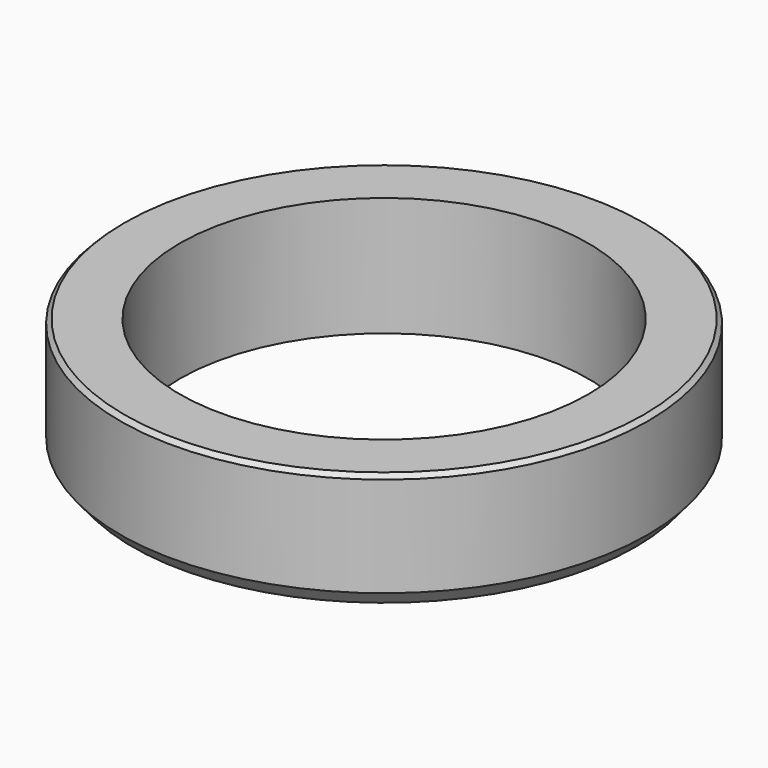
from build123d import *

# Parameters (mm, degrees)
F2_SIZE2 = 1.5748
F2_SIZE  = 1.5748
F4_DEPTH = 12.7
F5_R     = 76.2
F6_DEPTH = 44.451


with BuildPart() as f1:
    # F0 (on Front) → F1 (revolve)
    with BuildSketch(Plane.XZ):
        Polygon((98.425, 0), (0, 0), (0, -44.45), (93.726, -44.45), (98.425, -38.8499498684), align=None)
    revolve(axis=Axis((0, 0, -22.225), (0, 0, 1)))

    # F2
    f2_edges = [f1.edges().sort_by_distance(p)[0] for p in [
        (-98.425, 0, 0),
    ]]
    chamfer(f2_edges, length=F2_SIZE, length2=F2_SIZE2)

    # F3 (on face) → F4 (cut)
    with BuildSketch(Plane(origin=(0, 0, -44.45), x_dir=(1, 0, 0), z_dir=(0, 0, -1))):
        with BuildLine():
            ThreePointArc((59.6599475589, 65.9082745736), (59.7366637174, 59.7366637174), (65.9082745736, 59.6599475589))
            ThreePointArc((65.9082745736, 59.6599475589), (62.8617928475, 62.8617928475), (59.6599475589, 65.9082745736))
        make_face()
        with BuildLine():
            ThreePointArc((59.6599475589, 65.9082745736), (62.8617928475, 62.8617928475), (65.9082745736, 59.6599475589))
            ThreePointArc((65.9082745736, 59.6599475589), (66.923633243, 61.1198638129), (67.2813928475, 62.8617928475))
            ThreePointArc((67.2813928475, 62.8617928475), (64.5022179025, 66.9656775679), (59.6599475589, 65.9082745736))
        make_face()
        with BuildLine():
            ThreePointArc((90.2904059571, -23.0090131096), (89.343398088, -20.275157215), (86.9082138798, -18.7128928876))
            ThreePointArc((86.9082138798, -18.7128928876), (85.8708059571, -23.0090131096), (84.6211674612, -27.2482663209))
            ThreePointArc((84.6211674612, -27.2482663209), (88.5174984084, -26.5484881029), (90.2904059571, -23.0090131096))
        make_face()
        with BuildLine():
            ThreePointArc((84.6211674612, -27.2482663209), (85.8708059571, -23.0090131096), (86.9082138798, -18.7128928876))
            ThreePointArc((86.9082138798, -18.7128928876), (81.6018001752, -21.8651364579), (84.6211674612, -27.2482663209))
        make_face()
        with BuildLine():
            ThreePointArc((-18.5894131096, 85.8708059571), (-18.6203916237, 86.3931713593), (-18.7128928876, 86.9082138798))
            ThreePointArc((-18.7128928876, 86.9082138798), (-23.0090131096, 85.8708059571), (-27.2482663209, 84.6211674612))
            ThreePointArc((-27.2482663209, 84.6211674612), (-22.3777205201, 81.4965250075), (-18.5894131096, 85.8708059571))
        make_face()
        with BuildLine():
            ThreePointArc((-27.2482663209, 84.6211674612), (-23.0090131096, 85.8708059571), (-18.7128928876, 86.9082138798))
            ThreePointArc((-18.7128928876, 86.9082138798), (-24.1528897613, 90.139811739), (-27.2482663209, 84.6211674612))
        make_face()
        with BuildLine():
            ThreePointArc((27.4286131096, -85.8708059571), (27.3832940593, -85.2395133675), (27.2482663209, -84.6211674612))
            ThreePointArc((27.2482663209, -84.6211674612), (23.0090131096, -85.8708059571), (18.7128928876, -86.9082138798))
            ThreePointArc((18.7128928876, -86.9082138798), (23.5313785118, -90.259427443), (27.4286131096, -85.8708059571))
        make_face()
        with BuildLine():
            ThreePointArc((18.7128928876, -86.9082138798), (23.0090131096, -85.8708059571), (27.2482663209, -84.6211674612))
            ThreePointArc((27.2482663209, -84.6211674612), (21.8651364579, -81.6018001752), (18.7128928876, -86.9082138798))
        make_face()
        with BuildLine():
            ThreePointArc((-81.4512059571, 23.0090131096), (-82.3313309638, 25.6557055609), (-84.6211674612, 27.2482663209))
            ThreePointArc((-84.6211674612, 27.2482663209), (-85.8708059571, 23.0090131096), (-86.9082138798, 18.7128928876))
            ThreePointArc((-86.9082138798, 18.7128928876), (-83.1369500625, 19.5364209787), (-81.4512059571, 23.0090131096))
        make_face()
        with BuildLine():
            ThreePointArc((-86.9082138798, 18.7128928876), (-85.8708059571, 23.0090131096), (-84.6211674612, 27.2482663209))
            ThreePointArc((-84.6211674612, 27.2482663209), (-90.139811739, 24.1528897613), (-86.9082138798, 18.7128928876))
        make_face()
        with BuildLine():
            ThreePointArc((-65.9082745736, -59.6599475589), (-65.9869219776, -65.9869219776), (-59.6599475589, -65.9082745736))
            ThreePointArc((-59.6599475589, -65.9082745736), (-62.8617928475, -62.8617928475), (-65.9082745736, -59.6599475589))
        make_face()
        with BuildLine():
            ThreePointArc((-65.9082745736, -59.6599475589), (-62.8617928475, -62.8617928475), (-59.6599475589, -65.9082745736))
            ThreePointArc((-59.6599475589, -65.9082745736), (-58.757908127, -64.5022179025), (-58.4421928475, -62.8617928475))
            ThreePointArc((-58.4421928475, -62.8617928475), (-61.1198638129, -58.799952452), (-65.9082745736, -59.6599475589))
        make_face()
    extrude(amount=-F4_DEPTH, mode=Mode.SUBTRACT)

    # F5 (on face) → F6 (cut, through all)
    with BuildSketch(Plane.XY):
        Circle(F5_R)
    extrude(amount=-F6_DEPTH, mode=Mode.SUBTRACT)


solid = f1.part
